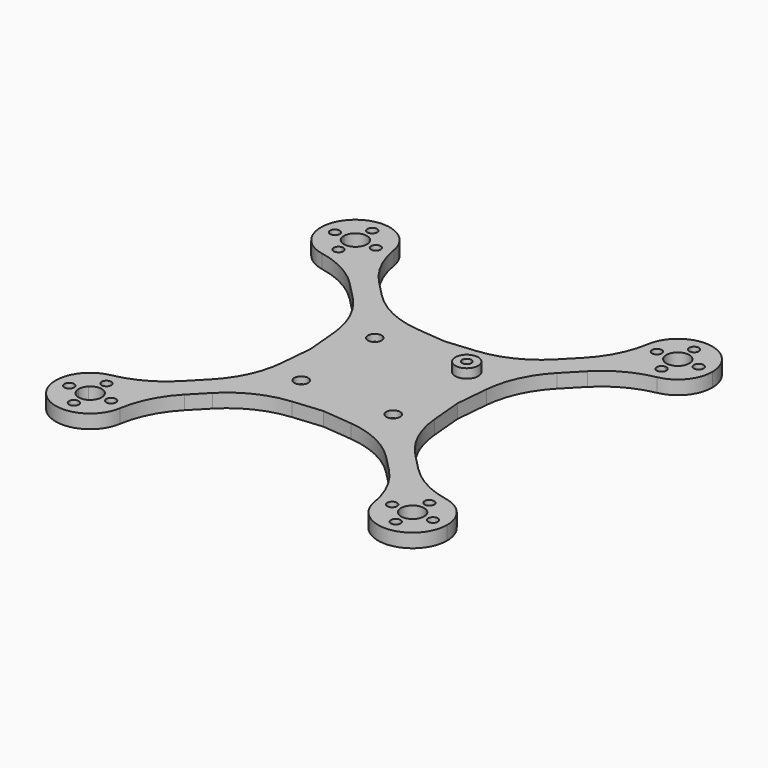
from build123d import *

# Parameters (mm, degrees)
F0_R      = 1.5
F0_R_2    = 1.05
F1_DEPTH  = 3
F2_R      = 20
F3_R      = 2.5
F4_DEPTH  = 1.5
F7_R      = 1.5
F7_R_2    = 1
F8_DEPTH  = 1.5
F9_R      = 2.5
F9_R_2    = 1.5
F9_R_3    = 1
F10_DEPTH = 2
F11_R     = 2.5
F11_R_2   = 1
F12_DEPTH = 2


with BuildPart() as f1:
    # F0 (on Top) → F1 (new body)
    with BuildSketch(Plane.XY):
        Polygon((17.5900963695, 18.0875221416), (13.7520964623, 17.7268610305), (0, 16.4345612622), (0, 0), (15.9825936427, 0), (17.239353816, 14.1409884306), align=None)
        with Locations((10, 10)):
            Circle(F0_R, mode=Mode.SUBTRACT)
        with BuildLine():
            ThreePointArc((31.9200670418, 29.2368537374), (29.8287845463, 30.6723050065), (28.3355882575, 32.722755607))
            Line((28.3355882575, 32.722755607), (13.7520964623, 17.7268610305))
            Line((13.7520964623, 17.7268610305), (17.5900963695, 18.0875221416))
            Line((17.5900963695, 18.0875221416), (17.239353816, 14.1409884306))
            Line((17.239353816, 14.1409884306), (31.9200670418, 29.2368537374))
        make_face()
        with BuildLine():
            ThreePointArc((31.9200670418, 29.2368537374), (39.1022771791, 29.7330997621), (42.5576373508, 36.049023183))
            ThreePointArc((42.5576373508, 36.049023183), (33.3496221576, 43.3519461663), (28.3355882575, 32.722755607))
            ThreePointArc((28.3355882575, 32.722755607), (29.8287845463, 30.6723050065), (31.9200670418, 29.2368537374))
        make_face()
        with BuildLine():
            ThreePointArc((35.1880737305, 32.5972755395), (35.8863959675, 32.2675873788), (36.1703713151, 31.5494604876))
            ThreePointArc((36.1703713151, 31.5494604876), (34.3543466627, 30.8313335964), (35.1880737305, 32.5972755395))
        make_face(mode=Mode.SUBTRACT)
        with Locations((30.5580746554, 35.9862892186)):
            Circle(F0_R_2, mode=Mode.SUBTRACT)
        with BuildLine():
            ThreePointArc((36.8498767429, 34.3060722482), (32.7413257914, 36.9896085113), (37.5576373508, 36.049023183))
            ThreePointArc((37.5576373508, 36.049023183), (37.3739489102, 35.1084378547), (36.8498767429, 34.3060722482))
        make_face(mode=Mode.SUBTRACT)
        with Locations((39.5572000461, 36.1117571474)):
            Circle(F0_R_2, mode=Mode.SUBTRACT)
        with Locations((34.9949033864, 40.5485858784)):
            Circle(F0_R_2, mode=Mode.SUBTRACT)
    extrude(amount=F1_DEPTH)

    # F2
    f2_edges = [f1.edges().sort_by_distance(p)[0] for p in [
        (17.239354, 14.140988, 1.5),
        (13.752096, 17.726861, 1.5),
        (31.920067, 29.236854, 1.5),
        (28.335588, 32.722756, 1.5),
    ]]
    fillet(f2_edges, radius=F2_R)

    # F3 (on face) → F4 (cut)
    with BuildSketch(Plane(origin=(0, 0, 0), x_dir=(1, 0, 0), z_dir=(0, 0, -1))):
        with Locations((10, -10)):
            Circle(F3_R)
    extrude(amount=-F4_DEPTH, mode=Mode.SUBTRACT)

    # F5: F1 across plane


with BuildPart() as f1_1:
    add(f1.part)
    add(f1.part.mirror(Plane.YZ))

    # F6: F1 across plane


with BuildPart() as f1_2:
    add(f1_1.part)
    add(f1_1.part.mirror(Plane.XZ))


with BuildPart() as f8:
    # F7 (on face) → F8 (new body)
    with BuildSketch(Plane.XY.offset(3)):
        with Locations((10, 10)):
            Circle(F7_R)
        with Locations((10, 10)):
            Circle(F7_R_2, mode=Mode.SUBTRACT)
    extrude(amount=-F8_DEPTH)

    # F9 (on face) → F10 (join)
    with BuildSketch(Plane(origin=(0, 0, 1.5), x_dir=(1, 0, 0), z_dir=(0, 0, -1))):
        with Locations((10, -10)):
            Circle(F9_R)
        with Locations((10, -10)):
            Circle(F9_R_2, mode=Mode.SUBTRACT)
        with Locations((10, -10)):
            Circle(F9_R_2)
        with Locations((10, -10)):
            Circle(F9_R_3, mode=Mode.SUBTRACT)
    extrude(amount=F10_DEPTH)

    # F11 (on face) → F12 (join)
    with BuildSketch(Plane.XY.offset(3)):
        with Locations((10, 10)):
            Circle(F11_R)
        with Locations((10, 10)):
            Circle(F11_R_2, mode=Mode.SUBTRACT)
    extrude(amount=F12_DEPTH)


solid = Compound([f1_2.part, f8.part])
